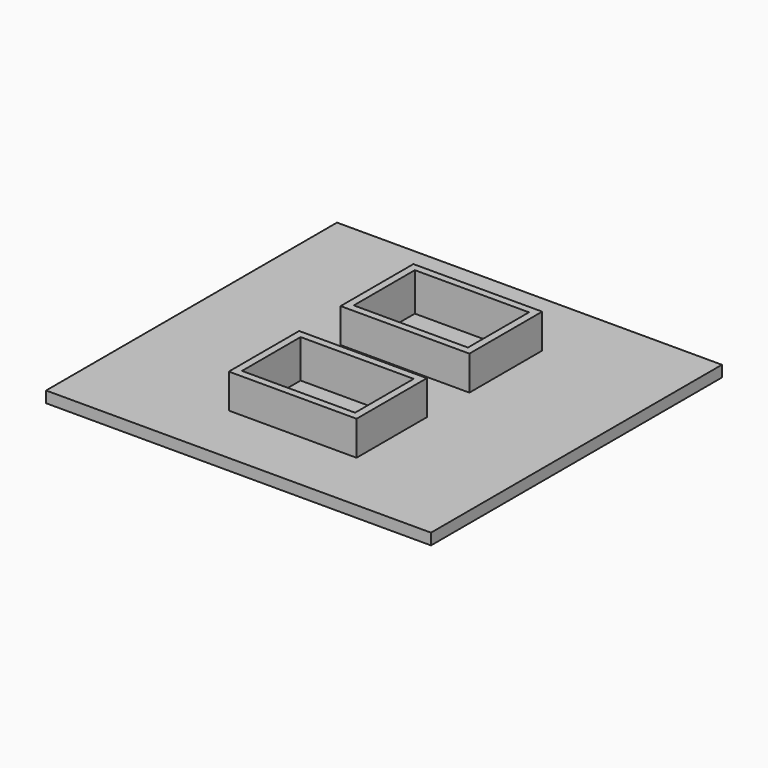
from build123d import *

# Parameters (mm, degrees)
F0_W        = 133.5890442133
F0_H        = 126.2129619718
F1_DEPTH    = 3.90208
F2_W        = 44.6898769587
F2_H        = 31.5666613169
F2_W_2      = 44.3351939321
F2_H_2      = 30.5026173592
F3_DEPTH    = 11.9221
F4_T        = 2.54
F4_T3_DEPTH = 49.4151939321
F4_T5_DEPTH = 35.5826173592
F4_T7_DEPTH = 49.7698769587
F4_T9_DEPTH = 36.6466613169


# Not quite as in the source:
# - a shell that OpenCascade refuses in one call is made with other operations: the cavity is built on its own and cut out


with BuildPart() as f1:
    # F0 (on Top) → F1 (new body)
    with BuildSketch(Plane.XY):
        with Locations((-0.6146728992, -2.3562498391)):
            Rectangle(F0_W, F0_H)
    extrude(amount=F1_DEPTH)

    # F2 (on face) → F3 (join)
    with BuildSketch(Plane.XY.offset(3.90208)):
        with Locations((0.623148866, 20.9897363093)):
            Rectangle(F2_W, F2_H)
        with Locations((0.8004903793, -28.4883454442)):
            Rectangle(F2_W_2, F2_H_2)
    extrude(amount=F3_DEPTH)

    # F4: shell of thickness 2.54, made by hand


with BuildPart() as f4_core1:
    # F4_t2: copy of F1
    add(f1.part)

    # the walls: a layer under each face that stays
    f4_faces = [f4_core1.faces().sort_by_distance(p)[0] for p in [
        (-0.6146728992, 60.7502311468, 1.95104),
        (66.1798492074, -2.3562498391, 1.95104),
        (-67.4091950059, -2.3562498391, 1.95104),
        (-0.6146728992, -2.3562498391, 0),
        (-0.6146728992, -2.3562498391, 3.90208),
        (-0.6146728992, -65.4627308249, 1.95104),
        (0.8004903793, -13.2370367646, 9.86313),
        (-21.3671065867, -28.4883454442, 9.86313),
        (0.8004903793, -43.7396541238, 9.86313),
        (22.9680873454, -28.4883454442, 9.86313),
        (0.623148866, 36.7730669677, 9.86313),
        (-21.7217896134, 20.9897363093, 9.86313),
        (0.623148866, 5.2064056508, 9.86313),
        (22.9680873454, 20.9897363093, 9.86313),
    ]]
    thicken(f4_faces, amount=-F4_T, mode=Mode.SUBTRACT)

    # F4_s4 → F4_t3 (cut)
    with BuildSketch(Plane.YZ.offset(-23.9071065867)):
        Polygon((-13.2116367646, 3.92748), (-13.2370367646, 1.36208), (-15.7770367646, 1.36208), (-15.7770367646, 3.90208), align=None)
        Polygon((-43.7650541238, 3.92748), (-43.7396541238, 1.36208), (-41.1996541238, 1.36208), (-41.1996541238, 3.90208), align=None)
    extrude(amount=F4_T3_DEPTH, mode=Mode.SUBTRACT)

    # F4_s6 → F4_t5 (cut)
    with BuildSketch(Plane.XZ.offset(10.6970367646)):
        Polygon((-21.3925065867, 3.92748), (-21.3671065867, 1.36208), (-18.8271065867, 1.36208), (-18.8271065867, 3.90208), align=None)
        Polygon((22.9934873454, 3.92748), (22.9680873454, 1.36208), (20.4280873454, 1.36208), (20.4280873454, 3.90208), align=None)
    extrude(amount=F4_T5_DEPTH, mode=Mode.SUBTRACT)

    # F4_s8 → F4_t7 (cut)
    with BuildSketch(Plane.YZ.offset(-24.2617896134)):
        Polygon((36.7984669677, 3.92748), (36.7730669677, 1.36208), (34.2330669677, 1.36208), (34.2330669677, 3.90208), align=None)
        Polygon((5.1810056508, 3.92748), (5.2064056508, 1.36208), (7.7464056508, 1.36208), (7.7464056508, 3.90208), align=None)
    extrude(amount=F4_T7_DEPTH, mode=Mode.SUBTRACT)

    # F4_s10 → F4_t9 (cut)
    with BuildSketch(Plane.XZ.offset(-39.3130669677)):
        Polygon((-21.7471896134, 3.92748), (-21.7217896134, 1.36208), (-19.1817896134, 1.36208), (-19.1817896134, 3.90208), align=None)
        Polygon((22.9934873454, 3.92748), (22.9680873454, 1.36208), (20.4280873454, 1.36208), (20.4280873454, 3.90208), align=None)
    extrude(amount=F4_T9_DEPTH, mode=Mode.SUBTRACT)


with BuildPart() as f1_1:
    add(f1.part)

    # what is left inside the walls is the cavity
    f4_cavity = [f4_core1.part.solids().sort_by_distance(p)[0] for p in [
        (0.80049, -32.725448, 2.5654),
        (0.623149, 16.575293, 2.5654),
    ]]
    add(f4_cavity, mode=Mode.SUBTRACT)


solid = f1_1.part
